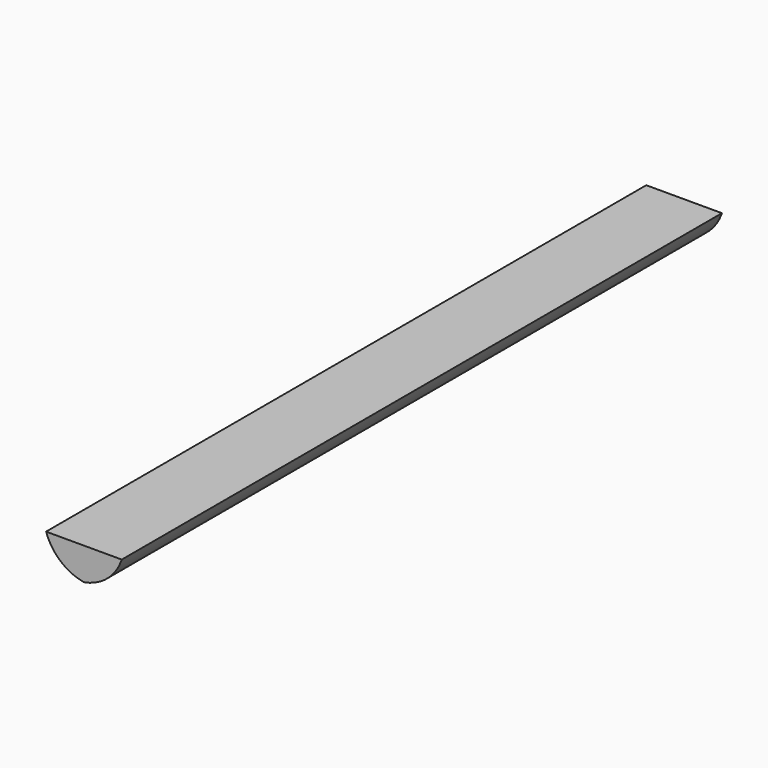
from build123d import *

# Parameters (mm, degrees)
F0_W        = 7.8275613487
F0_H        = 77.5999426842
F1_DEPTH    = 3.4
F2_T1_DEPTH = 101.2853812488


# Not quite as in the source:
# - a fillet or chamfer that OpenCascade refuses, or shapes differently, is made with other operations: its cross-section is extruded or revolved along the edge and cut away or added


with BuildPart() as f1:
    # F0 (on Top) → F1 (new body)
    with BuildSketch(Plane.XY):
        with Locations((-35.2240223438, 38.7999713421)):
            Rectangle(F0_W, F0_H)
    extrude(amount=F1_DEPTH)

    # F2: fillet of radius 5 on 2 edges, made by hand

    # F2_s2 → F2_t1 (cut)
    with BuildSketch(Plane.XZ.offset(-89.4426619665)):
        with BuildLine():
            ThreePointArc((-31.3102416694, 3.4), (-33.1318534349, 0.9379807977), (-36.0473293823, 0))
            Line((-36.0473293823, 0), (-31.3102416694, 0))
            Line((-31.3102416694, 0), (-31.3102416694, 3.4))
        make_face()
        with BuildLine():
            ThreePointArc((-39.1378030181, 3.4), (-37.3161912526, 0.9379807977), (-34.4007153052, 0))
            Line((-34.4007153052, 0), (-39.1378030181, 0))
            Line((-39.1378030181, 0), (-39.1378030181, 3.4))
        make_face()
    extrude(amount=F2_T1_DEPTH, mode=Mode.SUBTRACT)


solid = f1.part
